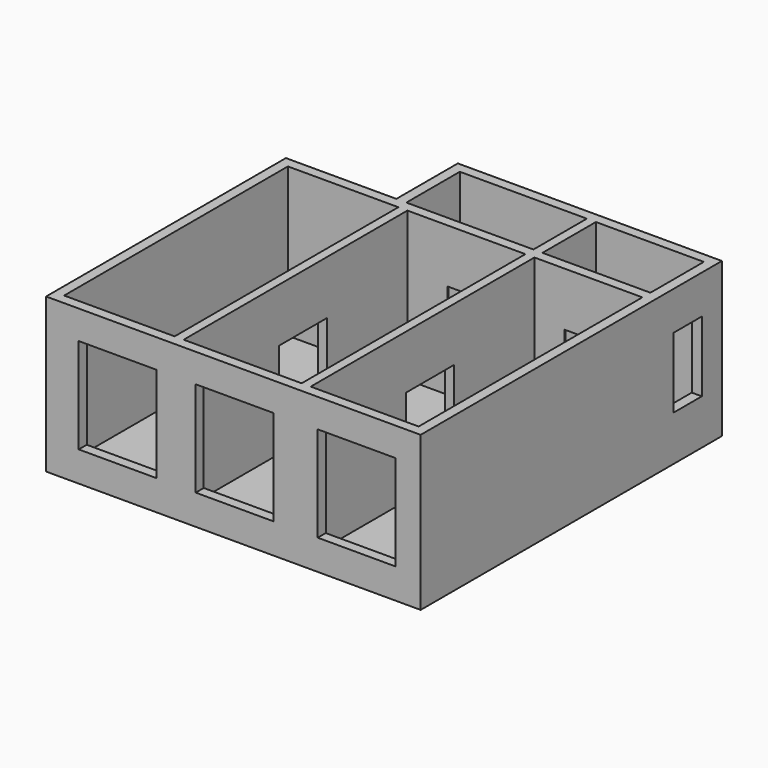
from build123d import *

# Parameters (mm, degrees)
F0_W           = 2200
F0_H           = 5570
F0_W_2         = 2350
F0_W_3         = 2150
F0_W_4         = 2530
F0_H_2         = 1330
F1_DEPTH       = 2970
F2_W           = 1550
F2_H           = 1900
F3_DEPTH       = 200
F4_W           = 700
F4_H           = 1400
F5_DEPTH       = 200
F7_DEPTH       = 100
F9_W           = 1200
F9_H           = 1900
F10_DEPTH      = 3000
F8_TEXT_SIZE   = 357.9835096995
F8_TEXT_SIZE_2 = 338.9626741409
F8_TEXT_SIZE_3 = 365.0618924035
F11_DEPTH      = 25
F12_W          = 800
F12_H          = 1900
F12_W_2        = 13.7615062607
F12_H_2        = 90.81533515
F12_W_3        = 16.1035829224
F12_H_3        = 106.2712360484
F12_H_4        = 150.8896411397
F13_DEPTH      = 25


# Not quite as in the source:
# - Text() gives the source's letters only with a copy of the font that has no kerning and outlines rounded to 1/6400 em; it was checked with that copy


with BuildPart() as f1:
    # F0 (on Top) → F1 (new body)
    with BuildSketch(Plane.XY):
        Polygon((200, 7300), (-5060, 7300), (-5060, 5770), (-7260, 5770), (-7260, -200), (200, -200), align=None)
        with Locations((-5960, 2785)):
            Rectangle(F0_W, F0_H, mode=Mode.SUBTRACT)
        with Locations((-3505, 2785)):
            Rectangle(F0_W_2, F0_H, mode=Mode.SUBTRACT)
        with Locations((-1075, 2785)):
            Rectangle(F0_W_3, F0_H, mode=Mode.SUBTRACT)
        with Locations((-3595, 6435)):
            Rectangle(F0_W_4, F0_H_2, mode=Mode.SUBTRACT)
        with Locations((-1075, 6435)):
            Rectangle(F0_W_3, F0_H_2, mode=Mode.SUBTRACT)
    extrude(amount=F1_DEPTH)

    # F2 (on face) → F3 (cut, through all)
    with BuildSketch(Plane(origin=(0, 0, 0), x_dir=(-1, 0, 0), z_dir=(0, 1, 0))):
        with Locations((1075, 1450)):
            Rectangle(F2_W, F2_H)
        with Locations((3505, 1450)):
            Rectangle(F2_W, F2_H)
        with Locations((5835, 1450)):
            Rectangle(F2_W, F2_H)
    extrude(amount=-F3_DEPTH, mode=Mode.SUBTRACT)

    # F4 (on face) → F5 (cut, through all)
    with BuildSketch(Plane(origin=(0, 0, 0), x_dir=(0, -1, 0), z_dir=(-1, 0, 0))):
        with Locations((-6450, 1500)):
            Rectangle(F4_W, F4_H)
    extrude(amount=-F5_DEPTH, mode=Mode.SUBTRACT)

    # F6 (on face) → F7 (join)
    with BuildSketch(Plane(origin=(0, 0, 0), x_dir=(1, 0, 0), z_dir=(0, 0, -1))):
        Polygon((200, 200), (-7260, 200), (-7260, -5770), (-5060, -5770), (-5060, -7300), (200, -7300), align=None)
    extrude(amount=F7_DEPTH)

    # F9 (on face) → F10 (cut)
    with BuildSketch(Plane(origin=(-4860, 0, 0), x_dir=(0, -1, 0), z_dir=(-1, 0, 0))):
        with Locations((-2970, 950)):
            Rectangle(F9_W, F9_H)
    extrude(amount=-F10_DEPTH, mode=Mode.SUBTRACT)

    # F8 (on face) → F11 (cut)
    with BuildSketch(Plane.XY):
        with Locations((-6638.8936042786, 3402.1844863892)):
            Text('Cuisine', F8_TEXT_SIZE, font='Open Sans', text_align=(TextAlign.LEFT, TextAlign.BOTTOM))
        with Locations((-6638.8936042786, 2915.3269131978)):
            Text('12m²', F8_TEXT_SIZE, font='Open Sans', text_align=(TextAlign.LEFT, TextAlign.BOTTOM))
        with Locations((-4455.9426307678, 3903.7611484528)):
            Text('salon', F8_TEXT_SIZE_2, font='Open Sans', text_align=(TextAlign.LEFT, TextAlign.BOTTOM))
        with Locations((-4455.9426307678, 3442.7719116211)):
            Text('12m²', F8_TEXT_SIZE_2, font='Open Sans', text_align=(TextAlign.LEFT, TextAlign.BOTTOM))
        with Locations((-4455.9426307678, 2520.7934379578)):
            Text('surface sans', F8_TEXT_SIZE_2, font='Open Sans', text_align=(TextAlign.LEFT, TextAlign.BOTTOM))
        with Locations((-4455.9426307678, 2059.8042011261)):
            Text('cloison 38m²', F8_TEXT_SIZE_2, font='Open Sans', text_align=(TextAlign.LEFT, TextAlign.BOTTOM))
        with Locations((-1840.2670621872, 3832.0169448853)):
            Text('chambre', F8_TEXT_SIZE_3, font='Open Sans', text_align=(TextAlign.LEFT, TextAlign.BOTTOM))
        with Locations((-1840.2670621872, 3335.5327712165)):
            Text('12m²', F8_TEXT_SIZE_3, font='Open Sans', text_align=(TextAlign.LEFT, TextAlign.BOTTOM))
    extrude(amount=-F11_DEPTH, mode=Mode.SUBTRACT)

    # F12 (on face) → F13 (cut)
    with BuildSketch(Plane.XZ.offset(-5570)):
        with Locations((-1150, 950)):
            Rectangle(F12_W, F12_H)
        with BuildLine():
            Line((-1405.2248319818, 966.460329377), (-1390.1375544051, 966.460329377))
            Line((-1390.1375544051, 966.460329377), (-1388.891329368, 964.5512186819))
            add(Edge.make_bspline(
                [(-1388.891329368, 964.5512186819), (-1391.0655943263, 956.2518902433), (-1395.1224545534, 945.2745037464)],
                knots=[0, 0, 0, 1, 1, 1], degree=2))
            add(Edge.make_bspline(
                [(-1395.1224545534, 945.2745037464), (-1399.1793147806, 934.2971172494), (-1403.5543601236, 924.8576254791)],
                knots=[0, 0, 0, 1, 1, 1], degree=2))
            Line((-1403.5543601236, 924.8576254791), (-1413.9218918151, 924.8576254791))
            add(Edge.make_bspline(
                [(-1413.9218918151, 924.8576254791), (-1411.6945960042, 933.4751390335), (-1409.0032802326, 946.149512815)],
                knots=[0, 0, 0, 1, 1, 1], degree=2))
            add(Edge.make_bspline(
                [(-1409.0032802326, 946.149512815), (-1406.311964461, 958.8238865965), (-1405.2248319818, 966.460329377)],
                knots=[0, 0, 0, 1, 1, 1], degree=2))
        make_face(mode=Mode.SUBTRACT)
        with BuildLine():
            add(Edge.make_bspline(
                [(-1442.5850676683, 1061.5313904515), (-1432.8008753558, 1053.4574431367), (-1432.8008753558, 1039.3777517602)],
                knots=[0, 0, 0, 1, 1, 1], degree=2))
            add(Edge.make_bspline(
                [(-1432.8008753558, 1039.3777517602), (-1432.8008753558, 1027.7639950315), (-1439.3104125176, 1020.3927065142)],
                knots=[0, 0, 0, 1, 1, 1], degree=2))
            add(Edge.make_bspline(
                [(-1439.3104125176, 1020.3927065142), (-1445.8199496795, 1013.0214179969), (-1457.751891524, 1010.5289679228)],
                knots=[0, 0, 0, 1, 1, 1], degree=2))
            Line((-1457.751891524, 1010.5289679228), (-1457.751891524, 1009.8660822647))
            add(Edge.make_bspline(
                [(-1457.751891524, 1009.8660822647), (-1443.1684070474, 1008.0630332749), (-1436.1285613591, 1000.5989407655)],
                knots=[0, 0, 0, 1, 1, 1], degree=2))
            add(Edge.make_bspline(
                [(-1436.1285613591, 1000.5989407655), (-1429.0887156708, 993.1348482561), (-1429.0887156708, 981.0438138536)],
                knots=[0, 0, 0, 1, 1, 1], degree=2))
            add(Edge.make_bspline(
                [(-1429.0887156708, 981.0438138536), (-1429.0887156708, 963.7292404659), (-1441.1002037943, 954.3958104009)],
                knots=[0, 0, 0, 1, 1, 1], degree=2))
            add(Edge.make_bspline(
                [(-1441.1002037943, 954.3958104009), (-1453.1116919178, 945.0623803358), (-1475.2255574697, 945.0623803358)],
                knots=[0, 0, 0, 1, 1, 1], degree=2))
            add(Edge.make_bspline(
                [(-1475.2255574697, 945.0623803358), (-1484.8506572242, 945.0623803358), (-1492.8450582601, 946.5207287835)],
                knots=[0, 0, 0, 1, 1, 1], degree=2))
            add(Edge.make_bspline(
                [(-1492.8450582601, 946.5207287835), (-1500.8394592959, 947.9790772311), (-1508.3698403711, 951.6116906371)],
                knots=[0, 0, 0, 1, 1, 1], degree=2))
            Line((-1508.3698403711, 951.6116906371), (-1508.3698403711, 964.7103112398))
            add(Edge.make_bspline(
                [(-1508.3698403711, 964.7103112398), (-1500.4947587537, 960.8125435706), (-1491.5855755098, 958.784113457)],
                knots=[0, 0, 0, 1, 1, 1], degree=2))
            add(Edge.make_bspline(
                [(-1491.5855755098, 958.784113457), (-1482.6763922659, 956.7556833434), (-1474.7217643696, 956.7556833434)],
                knots=[0, 0, 0, 1, 1, 1], degree=2))
            add(Edge.make_bspline(
                [(-1474.7217643696, 956.7556833434), (-1443.3274996053, 956.7556833434), (-1443.3274996053, 981.3619989695)],
                knots=[0, 0, 0, 1, 1, 1], degree=2))
            add(Edge.make_bspline(
                [(-1443.3274996053, 981.3619989695), (-1443.3274996053, 1003.4228336687), (-1477.9566463807, 1003.4228336687)],
                knots=[0, 0, 0, 1, 1, 1], degree=2))
            Line((-1477.9566463807, 1003.4228336687), (-1489.8885882253, 1003.4228336687))
            Line((-1489.8885882253, 1003.4228336687), (-1489.8885882253, 1015.2487138079))
            Line((-1489.8885882253, 1015.2487138079), (-1477.7975538228, 1015.2487138079))
            add(Edge.make_bspline(
                [(-1477.7975538228, 1015.2487138079), (-1463.6383161673, 1015.2487138079), (-1455.3522454419, 1021.5063544197)],
                knots=[0, 0, 0, 1, 1, 1], degree=2))
            add(Edge.make_bspline(
                [(-1455.3522454419, 1021.5063544197), (-1447.0661747166, 1027.7639950315), (-1447.0661747166, 1038.8739586601)],
                knots=[0, 0, 0, 1, 1, 1], degree=2))
            add(Edge.make_bspline(
                [(-1447.0661747166, 1038.8739586601), (-1447.0661747166, 1047.7301110514), (-1453.1514650573, 1052.7945574787)],
                knots=[0, 0, 0, 1, 1, 1], degree=2))
            add(Edge.make_bspline(
                [(-1453.1514650573, 1052.7945574787), (-1459.236755398, 1057.859003906), (-1469.6838333685, 1057.859003906)],
                knots=[0, 0, 0, 1, 1, 1], degree=2))
            add(Edge.make_bspline(
                [(-1469.6838333685, 1057.859003906), (-1477.6384612649, 1057.859003906), (-1484.6783069532, 1055.6979966609)],
                knots=[0, 0, 0, 1, 1, 1], degree=2))
            add(Edge.make_bspline(
                [(-1484.6783069532, 1055.6979966609), (-1491.7181526414, 1053.5369894157), (-1500.7599130169, 1047.7301110514)],
                knots=[0, 0, 0, 1, 1, 1], degree=2))
            Line((-1500.7599130169, 1047.7301110514), (-1507.7069547131, 1057.0105102638))
            add(Edge.make_bspline(
                [(-1507.7069547131, 1057.0105102638), (-1500.2561199168, 1062.8969349071), (-1490.524958457, 1066.2511363367)],
                knots=[0, 0, 0, 1, 1, 1], degree=2))
            add(Edge.make_bspline(
                [(-1490.524958457, 1066.2511363367), (-1480.7937969971, 1069.6053377663), (-1470.0020184844, 1069.6053377663)],
                knots=[0, 0, 0, 1, 1, 1], degree=2))
            add(Edge.make_bspline(
                [(-1470.0020184844, 1069.6053377663), (-1452.3692599808, 1069.6053377663), (-1442.5850676683, 1061.5313904515)],
                knots=[0, 0, 0, 1, 1, 1], degree=2))
        make_face(mode=Mode.SUBTRACT)
        with BuildLine():
            add(Edge.make_bspline(
                [(-1303.9624188613, 1061.5313904515), (-1294.1782265488, 1053.4574431367), (-1294.1782265488, 1039.3777517602)],
                knots=[0, 0, 0, 1, 1, 1], degree=2))
            add(Edge.make_bspline(
                [(-1294.1782265488, 1039.3777517602), (-1294.1782265488, 1027.7639950315), (-1300.6877637106, 1020.3927065142)],
                knots=[0, 0, 0, 1, 1, 1], degree=2))
            add(Edge.make_bspline(
                [(-1300.6877637106, 1020.3927065142), (-1307.1973008725, 1013.0214179969), (-1319.129242717, 1010.5289679228)],
                knots=[0, 0, 0, 1, 1, 1], degree=2))
            Line((-1319.129242717, 1010.5289679228), (-1319.129242717, 1009.8660822647))
            add(Edge.make_bspline(
                [(-1319.129242717, 1009.8660822647), (-1304.5457582403, 1008.0630332749), (-1297.5059125521, 1000.5989407655)],
                knots=[0, 0, 0, 1, 1, 1], degree=2))
            add(Edge.make_bspline(
                [(-1297.5059125521, 1000.5989407655), (-1290.4660668638, 993.1348482561), (-1290.4660668638, 981.0438138536)],
                knots=[0, 0, 0, 1, 1, 1], degree=2))
            add(Edge.make_bspline(
                [(-1290.4660668638, 981.0438138536), (-1290.4660668638, 963.7292404659), (-1302.4775549873, 954.3958104009)],
                knots=[0, 0, 0, 1, 1, 1], degree=2))
            add(Edge.make_bspline(
                [(-1302.4775549873, 954.3958104009), (-1314.4890431108, 945.0623803358), (-1336.6029086626, 945.0623803358)],
                knots=[0, 0, 0, 1, 1, 1], degree=2))
            add(Edge.make_bspline(
                [(-1336.6029086626, 945.0623803358), (-1346.2280084172, 945.0623803358), (-1354.222409453, 946.5207287835)],
                knots=[0, 0, 0, 1, 1, 1], degree=2))
            add(Edge.make_bspline(
                [(-1354.222409453, 946.5207287835), (-1362.2168104889, 947.9790772311), (-1369.7471915641, 951.6116906371)],
                knots=[0, 0, 0, 1, 1, 1], degree=2))
            Line((-1369.7471915641, 951.6116906371), (-1369.7471915641, 964.7103112398))
            add(Edge.make_bspline(
                [(-1369.7471915641, 964.7103112398), (-1361.8721099467, 960.8125435706), (-1352.9629267028, 958.784113457)],
                knots=[0, 0, 0, 1, 1, 1], degree=2))
            add(Edge.make_bspline(
                [(-1352.9629267028, 958.784113457), (-1344.0537434589, 956.7556833434), (-1336.0991155625, 956.7556833434)],
                knots=[0, 0, 0, 1, 1, 1], degree=2))
            add(Edge.make_bspline(
                [(-1336.0991155625, 956.7556833434), (-1304.7048507983, 956.7556833434), (-1304.7048507983, 981.3619989695)],
                knots=[0, 0, 0, 1, 1, 1], degree=2))
            add(Edge.make_bspline(
                [(-1304.7048507983, 981.3619989695), (-1304.7048507983, 1003.4228336687), (-1339.3339975737, 1003.4228336687)],
                knots=[0, 0, 0, 1, 1, 1], degree=2))
            Line((-1339.3339975737, 1003.4228336687), (-1351.2659394182, 1003.4228336687))
            Line((-1351.2659394182, 1003.4228336687), (-1351.2659394182, 1015.2487138079))
            Line((-1351.2659394182, 1015.2487138079), (-1339.1749050158, 1015.2487138079))
            add(Edge.make_bspline(
                [(-1339.1749050158, 1015.2487138079), (-1325.0156673603, 1015.2487138079), (-1316.7295966349, 1021.5063544197)],
                knots=[0, 0, 0, 1, 1, 1], degree=2))
            add(Edge.make_bspline(
                [(-1316.7295966349, 1021.5063544197), (-1308.4435259095, 1027.7639950315), (-1308.4435259095, 1038.8739586601)],
                knots=[0, 0, 0, 1, 1, 1], degree=2))
            add(Edge.make_bspline(
                [(-1308.4435259095, 1038.8739586601), (-1308.4435259095, 1047.7301110514), (-1314.5288162503, 1052.7945574787)],
                knots=[0, 0, 0, 1, 1, 1], degree=2))
            add(Edge.make_bspline(
                [(-1314.5288162503, 1052.7945574787), (-1320.614106591, 1057.859003906), (-1331.0611845615, 1057.859003906)],
                knots=[0, 0, 0, 1, 1, 1], degree=2))
            add(Edge.make_bspline(
                [(-1331.0611845615, 1057.859003906), (-1339.0158124578, 1057.859003906), (-1346.0556581461, 1055.6979966609)],
                knots=[0, 0, 0, 1, 1, 1], degree=2))
            add(Edge.make_bspline(
                [(-1346.0556581461, 1055.6979966609), (-1353.0955038344, 1053.5369894157), (-1362.1372642099, 1047.7301110514)],
                knots=[0, 0, 0, 1, 1, 1], degree=2))
            Line((-1362.1372642099, 1047.7301110514), (-1369.084305906, 1057.0105102638))
            add(Edge.make_bspline(
                [(-1369.084305906, 1057.0105102638), (-1361.6334711098, 1062.8969349071), (-1351.9023096499, 1066.2511363367)],
                knots=[0, 0, 0, 1, 1, 1], degree=2))
            add(Edge.make_bspline(
                [(-1351.9023096499, 1066.2511363367), (-1342.1711481901, 1069.6053377663), (-1331.3793696774, 1069.6053377663)],
                knots=[0, 0, 0, 1, 1, 1], degree=2))
            add(Edge.make_bspline(
                [(-1331.3793696774, 1069.6053377663), (-1313.7466111738, 1069.6053377663), (-1303.9624188613, 1061.5313904515)],
                knots=[0, 0, 0, 1, 1, 1], degree=2))
        make_face(mode=Mode.SUBTRACT)
        with BuildLine():
            Line((-1136.4379553642, 946.732852194), (-1150.1729461985, 946.732852194))
            Line((-1150.1729461985, 946.732852194), (-1150.1729461985, 1005.8092220376))
            add(Edge.make_bspline(
                [(-1150.1729461985, 1005.8092220376), (-1150.1729461985, 1016.6805468293), (-1154.8131458047, 1022.1029515119)],
                knots=[0, 0, 0, 1, 1, 1], degree=2))
            add(Edge.make_bspline(
                [(-1154.8131458047, 1022.1029515119), (-1159.4533454109, 1027.5253561946), (-1169.2375377234, 1027.5253561946)],
                knots=[0, 0, 0, 1, 1, 1], degree=2))
            add(Edge.make_bspline(
                [(-1169.2375377234, 1027.5253561946), (-1182.0710040629, 1027.5253561946), (-1188.2093252562, 1020.1540676773)],
                knots=[0, 0, 0, 1, 1, 1], degree=2))
            add(Edge.make_bspline(
                [(-1188.2093252562, 1020.1540676773), (-1194.3476464496, 1012.7827791601), (-1194.3476464496, 997.4568627464)],
                knots=[0, 0, 0, 1, 1, 1], degree=2))
            Line((-1194.3476464496, 997.4568627464), (-1194.3476464496, 946.732852194))
            Line((-1194.3476464496, 946.732852194), (-1208.1091527103, 946.732852194))
            Line((-1208.1091527103, 946.732852194), (-1208.1091527103, 1005.8092220376))
            add(Edge.make_bspline(
                [(-1208.1091527103, 1005.8092220376), (-1208.1091527103, 1016.6805468293), (-1212.7493523165, 1022.1029515119)],
                knots=[0, 0, 0, 1, 1, 1], degree=2))
            add(Edge.make_bspline(
                [(-1212.7493523165, 1022.1029515119), (-1217.3895519227, 1027.5253561946), (-1227.2532905142, 1027.5253561946)],
                knots=[0, 0, 0, 1, 1, 1], degree=2))
            add(Edge.make_bspline(
                [(-1227.2532905142, 1027.5253561946), (-1240.1663031326, 1027.5253561946), (-1246.1720471943, 1019.7828517088)],
                knots=[0, 0, 0, 1, 1, 1], degree=2))
            add(Edge.make_bspline(
                [(-1246.1720471943, 1019.7828517088), (-1252.177791256, 1012.0403472231), (-1252.177791256, 994.3810732932)],
                knots=[0, 0, 0, 1, 1, 1], degree=2))
            Line((-1252.177791256, 994.3810732932), (-1252.177791256, 946.732852194))
            Line((-1252.177791256, 946.732852194), (-1265.9392975167, 946.732852194))
            Line((-1265.9392975167, 946.732852194), (-1265.9392975167, 1037.548187344))
            Line((-1265.9392975167, 1037.548187344), (-1254.7497876092, 1037.548187344))
            Line((-1254.7497876092, 1037.548187344), (-1252.5224917982, 1025.1124523994))
            Line((-1252.5224917982, 1025.1124523994), (-1251.8596061402, 1025.1124523994))
            add(Edge.make_bspline(
                [(-1251.8596061402, 1025.1124523994), (-1247.961838471, 1031.7413089797), (-1240.8689619301, 1035.479984091)],
                knots=[0, 0, 0, 1, 1, 1], degree=2))
            add(Edge.make_bspline(
                [(-1240.8689619301, 1035.479984091), (-1233.7760853892, 1039.2186592023), (-1224.9994792769, 1039.2186592023)],
                knots=[0, 0, 0, 1, 1, 1], degree=2))
            add(Edge.make_bspline(
                [(-1224.9994792769, 1039.2186592023), (-1203.707591941, 1039.2186592023), (-1197.1582816396, 1023.7866810833)],
                knots=[0, 0, 0, 1, 1, 1], degree=2))
            Line((-1197.1582816396, 1023.7866810833), (-1196.4953959816, 1023.7866810833))
            add(Edge.make_bspline(
                [(-1196.4953959816, 1023.7866810833), (-1192.4385357545, 1030.9193307637), (-1184.7358044082, 1035.068994983)],
                knots=[0, 0, 0, 1, 1, 1], degree=2))
            add(Edge.make_bspline(
                [(-1184.7358044082, 1035.068994983), (-1177.0330730619, 1039.2186592023), (-1167.1693344704, 1039.2186592023)],
                knots=[0, 0, 0, 1, 1, 1], degree=2))
            add(Edge.make_bspline(
                [(-1167.1693344704, 1039.2186592023), (-1151.7638717778, 1039.2186592023), (-1144.100913571, 1031.3038044454)],
                knots=[0, 0, 0, 1, 1, 1], degree=2))
            add(Edge.make_bspline(
                [(-1144.100913571, 1031.3038044454), (-1136.4379553642, 1023.3889496885), (-1136.4379553642, 1005.9683145955)],
                knots=[0, 0, 0, 1, 1, 1], degree=2))
            Line((-1136.4379553642, 1005.9683145955), (-1136.4379553642, 946.732852194))
        make_face(mode=Mode.SUBTRACT)
        with BuildLine():
            Line((-1068.558463982, 1005.1463363796), (-1068.558463982, 995.2825977881))
            Line((-1068.558463982, 995.2825977881), (-1118.6195888764, 995.2825977881))
            Line((-1118.6195888764, 995.2825977881), (-1118.6195888764, 1003.9001113425))
            Line((-1118.6195888764, 1003.9001113425), (-1099.0512042513, 1022.9647028674))
            add(Edge.make_bspline(
                [(-1099.0512042513, 1022.9647028674), (-1091.679915734, 1030.0973525478), (-1088.2859411649, 1034.1144396354)],
                knots=[0, 0, 0, 1, 1, 1], degree=2))
            add(Edge.make_bspline(
                [(-1088.2859411649, 1034.1144396354), (-1084.8919665958, 1038.1315267231), (-1083.5264221403, 1041.2736047421)],
                knots=[0, 0, 0, 1, 1, 1], degree=2))
            add(Edge.make_bspline(
                [(-1083.5264221403, 1041.2736047421), (-1082.1608776848, 1044.4156827612), (-1082.1608776848, 1048.8967898095)],
                knots=[0, 0, 0, 1, 1, 1], degree=2))
            add(Edge.make_bspline(
                [(-1082.1608776848, 1048.8967898095), (-1082.1608776848, 1054.5445756159), (-1085.4753059749, 1057.3949839454)],
                knots=[0, 0, 0, 1, 1, 1], degree=2))
            add(Edge.make_bspline(
                [(-1085.4753059749, 1057.3949839454), (-1088.789734265, 1060.2453922749), (-1094.0132732503, 1060.2453922749)],
                knots=[0, 0, 0, 1, 1, 1], degree=2))
            add(Edge.make_bspline(
                [(-1094.0132732503, 1060.2453922749), (-1098.3087723143, 1060.2453922749), (-1102.3656325415, 1058.680982122)],
                knots=[0, 0, 0, 1, 1, 1], degree=2))
            add(Edge.make_bspline(
                [(-1102.3656325415, 1058.680982122), (-1106.4224927686, 1057.116571969), (-1112.149824854, 1052.9536500366)],
                knots=[0, 0, 0, 1, 1, 1], degree=2))
            Line((-1112.149824854, 1052.9536500366), (-1117.6120026761, 1060.2453922749))
            add(Edge.make_bspline(
                [(-1117.6120026761, 1060.2453922749), (-1106.7671933108, 1069.4462452084), (-1094.1723658082, 1069.4462452084)],
                knots=[0, 0, 0, 1, 1, 1], degree=2))
            add(Edge.make_bspline(
                [(-1094.1723658082, 1069.4462452084), (-1083.2214947376, 1069.4462452084), (-1077.1362043969, 1064.0636136652)],
                knots=[0, 0, 0, 1, 1, 1], degree=2))
            add(Edge.make_bspline(
                [(-1077.1362043969, 1064.0636136652), (-1071.0509140562, 1058.680982122), (-1071.0509140562, 1049.4005829096)],
                knots=[0, 0, 0, 1, 1, 1], degree=2))
            add(Edge.make_bspline(
                [(-1071.0509140562, 1049.4005829096), (-1071.0509140562, 1042.7717263293), (-1074.7365583148, 1036.5140857175)],
                knots=[0, 0, 0, 1, 1, 1], degree=2))
            add(Edge.make_bspline(
                [(-1074.7365583148, 1036.5140857175), (-1078.4222025735, 1030.2564451057), (-1090.6192986812, 1018.8282963613)],
                knots=[0, 0, 0, 1, 1, 1], degree=2))
            Line((-1090.6192986812, 1018.8282963613), (-1105.0171751736, 1005.1463363796))
            Line((-1105.0171751736, 1005.1463363796), (-1068.558463982, 1005.1463363796))
        make_face(mode=Mode.SUBTRACT)
        with BuildLine():
            add(Edge.make_bspline(
                [(-1487.8203849722, 1256.247423641), (-1478.221800644, 1269.8233219174), (-1459.316301677, 1269.8233219174)],
                knots=[0, 0, 0, 1, 1, 1], degree=2))
            add(Edge.make_bspline(
                [(-1459.316301677, 1269.8233219174), (-1441.4183889102, 1269.8233219174), (-1431.5148771792, 1257.5997103833)],
                knots=[0, 0, 0, 1, 1, 1], degree=2))
            add(Edge.make_bspline(
                [(-1431.5148771792, 1257.5997103833), (-1421.6113654483, 1245.3760988493), (-1421.6113654483, 1223.0235944606)],
                knots=[0, 0, 0, 1, 1, 1], degree=2))
            add(Edge.make_bspline(
                [(-1421.6113654483, 1223.0235944606), (-1421.6113654483, 1200.6445746455), (-1431.5944234582, 1188.2486128403)],
                knots=[0, 0, 0, 1, 1, 1], degree=2))
            add(Edge.make_bspline(
                [(-1431.5944234582, 1188.2486128403), (-1441.5774814681, 1175.8526510352), (-1459.316301677, 1175.8526510352)],
                knots=[0, 0, 0, 1, 1, 1], degree=2))
            add(Edge.make_bspline(
                [(-1459.316301677, 1175.8526510352), (-1468.1989694946, 1175.8526510352), (-1475.5304848724, 1179.1273061859)],
                knots=[0, 0, 0, 1, 1, 1], degree=2))
            add(Edge.make_bspline(
                [(-1475.5304848724, 1179.1273061859), (-1482.8620002502, 1182.4019613365), (-1487.8203849722, 1189.2164259011)],
                knots=[0, 0, 0, 1, 1, 1], degree=2))
            Line((-1487.8203849722, 1189.2164259011), (-1488.8279711724, 1189.2164259011))
            Line((-1488.8279711724, 1189.2164259011), (-1491.7181526414, 1177.5231228934))
            Line((-1491.7181526414, 1177.5231228934), (-1501.5818912329, 1177.5231228934))
            Line((-1501.5818912329, 1177.5231228934), (-1501.5818912329, 1306.4676410933))
            Line((-1501.5818912329, 1306.4676410933), (-1487.8203849722, 1306.4676410933))
            Line((-1487.8203849722, 1306.4676410933), (-1487.8203849722, 1275.1264071816))
            add(Edge.make_bspline(
                [(-1487.8203849722, 1275.1264071816), (-1487.8203849722, 1264.5997829321), (-1488.4832706302, 1256.247423641)],
                knots=[0, 0, 0, 1, 1, 1], degree=2))
            Line((-1488.4832706302, 1256.247423641), (-1487.8203849722, 1256.247423641))
        make_face(mode=Mode.SUBTRACT)
        with BuildLine():
            Line((-1331.5384622353, 1177.5231228934), (-1341.7469013689, 1177.5231228934))
            Line((-1341.7469013689, 1177.5231228934), (-1344.47799028, 1190.4626509382))
            Line((-1344.47799028, 1190.4626509382), (-1345.140875938, 1190.4626509382))
            add(Edge.make_bspline(
                [(-1345.140875938, 1190.4626509382), (-1351.9288250763, 1181.9246836628), (-1358.677001075, 1178.888667349)],
                knots=[0, 0, 0, 1, 1, 1], degree=2))
            add(Edge.make_bspline(
                [(-1358.677001075, 1178.888667349), (-1365.4251770737, 1175.8526510352), (-1375.5540699284, 1175.8526510352)],
                knots=[0, 0, 0, 1, 1, 1], degree=2))
            add(Edge.make_bspline(
                [(-1375.5540699284, 1175.8526510352), (-1389.0504219259, 1175.8526510352), (-1396.7133801327, 1182.8262081577)],
                knots=[0, 0, 0, 1, 1, 1], degree=2))
            add(Edge.make_bspline(
                [(-1396.7133801327, 1182.8262081577), (-1404.3763383395, 1189.7997652801), (-1404.3763383395, 1202.6332316196)],
                knots=[0, 0, 0, 1, 1, 1], degree=2))
            add(Edge.make_bspline(
                [(-1404.3763383395, 1202.6332316196), (-1404.3763383395, 1230.1297287146), (-1360.3872460727, 1231.4555000307)],
                knots=[0, 0, 0, 1, 1, 1], degree=2))
            Line((-1360.3872460727, 1231.4555000307), (-1344.9817833801, 1231.9592931308))
            Line((-1344.9817833801, 1231.9592931308), (-1344.9817833801, 1237.6070789372))
            add(Edge.make_bspline(
                [(-1344.9817833801, 1237.6070789372), (-1344.9817833801, 1248.2927957446), (-1349.5689521337, 1253.3837575983)],
                knots=[0, 0, 0, 1, 1, 1], degree=2))
            add(Edge.make_bspline(
                [(-1349.5689521337, 1253.3837575983), (-1354.1561208872, 1258.4747194519), (-1364.2850137419, 1258.4747194519)],
                knots=[0, 0, 0, 1, 1, 1], degree=2))
            add(Edge.make_bspline(
                [(-1364.2850137419, 1258.4747194519), (-1375.6336162074, 1258.4747194519), (-1389.9519464208, 1251.5276777558)],
                knots=[0, 0, 0, 1, 1, 1], degree=2))
            Line((-1389.9519464208, 1251.5276777558), (-1394.1944146322, 1262.0543020053))
            add(Edge.make_bspline(
                [(-1394.1944146322, 1262.0543020053), (-1387.4860117729, 1265.6869154113), (-1379.4916107371, 1267.7551186644)],
                knots=[0, 0, 0, 1, 1, 1], degree=2))
            add(Edge.make_bspline(
                [(-1379.4916107371, 1267.7551186644), (-1371.4972097013, 1269.8233219174), (-1363.4365200996, 1269.8233219174)],
                knots=[0, 0, 0, 1, 1, 1], degree=2))
            add(Edge.make_bspline(
                [(-1363.4365200996, 1269.8233219174), (-1347.2090791911, 1269.8233219174), (-1339.3737707132, 1262.6243836712)],
                knots=[0, 0, 0, 1, 1, 1], degree=2))
            add(Edge.make_bspline(
                [(-1339.3737707132, 1262.6243836712), (-1331.5384622353, 1255.425445425), (-1331.5384622353, 1239.5161896323)],
                knots=[0, 0, 0, 1, 1, 1], degree=2))
            Line((-1331.5384622353, 1239.5161896323), (-1331.5384622353, 1177.5231228934))
        make_face(mode=Mode.SUBTRACT)
        with Locations((-1296.3392337939, 1222.9307904684)):
            Rectangle(F12_W_2, F12_H_2, mode=Mode.SUBTRACT)
        with BuildLine():
            Line((-1217.3630364964, 1268.3384580434), (-1185.9687717321, 1268.3384580434))
            Line((-1185.9687717321, 1268.3384580434), (-1185.9687717321, 1259.6413982101))
            Line((-1185.9687717321, 1259.6413982101), (-1202.7795520197, 1257.652741236))
            add(Edge.make_bspline(
                [(-1202.7795520197, 1257.652741236), (-1200.4727099298, 1254.762559767), (-1198.6431455136, 1250.0693293081)],
                knots=[0, 0, 0, 1, 1, 1], degree=2))
            add(Edge.make_bspline(
                [(-1198.6431455136, 1250.0693293081), (-1196.8135810975, 1245.3760988493), (-1196.8135810975, 1239.5161896323)],
                knots=[0, 0, 0, 1, 1, 1], degree=2))
            add(Edge.make_bspline(
                [(-1196.8135810975, 1239.5161896323), (-1196.8135810975, 1226.1524147665), (-1205.9348877519, 1218.1977868701)],
                knots=[0, 0, 0, 1, 1, 1], degree=2))
            add(Edge.make_bspline(
                [(-1205.9348877519, 1218.1977868701), (-1215.0561944064, 1210.2431589738), (-1230.9654501991, 1210.2431589738)],
                knots=[0, 0, 0, 1, 1, 1], degree=2))
            add(Edge.make_bspline(
                [(-1230.9654501991, 1210.2431589738), (-1235.0223104263, 1210.2431589738), (-1238.5753775533, 1210.9060446318)],
                knots=[0, 0, 0, 1, 1, 1], degree=2))
            add(Edge.make_bspline(
                [(-1238.5753775533, 1210.9060446318), (-1247.3519836656, 1206.2658450256), (-1247.3519836656, 1199.2392570505)],
                knots=[0, 0, 0, 1, 1, 1], degree=2))
            add(Edge.make_bspline(
                [(-1247.3519836656, 1199.2392570505), (-1247.3519836656, 1195.5005819392), (-1244.2894519255, 1193.7240483757)],
                knots=[0, 0, 0, 1, 1, 1], degree=2))
            add(Edge.make_bspline(
                [(-1244.2894519255, 1193.7240483757), (-1241.2269201854, 1191.9475148122), (-1233.7760853892, 1191.9475148122)],
                knots=[0, 0, 0, 1, 1, 1], degree=2))
            Line((-1233.7760853892, 1191.9475148122), (-1217.7077370385, 1191.9475148122))
            add(Edge.make_bspline(
                [(-1217.7077370385, 1191.9475148122), (-1202.9386445776, 1191.9475148122), (-1195.0370475339, 1185.7296473398)],
                knots=[0, 0, 0, 1, 1, 1], degree=2))
            add(Edge.make_bspline(
                [(-1195.0370475339, 1185.7296473398), (-1187.1354504902, 1179.5117798675), (-1187.1354504902, 1167.659384302)],
                knots=[0, 0, 0, 1, 1, 1], degree=2))
            add(Edge.make_bspline(
                [(-1187.1354504902, 1167.659384302), (-1187.1354504902, 1152.5721067252), (-1199.2264848927, 1144.6572519684)],
                knots=[0, 0, 0, 1, 1, 1], degree=2))
            add(Edge.make_bspline(
                [(-1199.2264848927, 1144.6572519684), (-1211.3175192951, 1136.7423972115), (-1234.5185173261, 1136.7423972115)],
                knots=[0, 0, 0, 1, 1, 1], degree=2))
            add(Edge.make_bspline(
                [(-1234.5185173261, 1136.7423972115), (-1252.336883814, 1136.7423972115), (-1261.9884989949, 1143.3712537918)],
                knots=[0, 0, 0, 1, 1, 1], degree=2))
            add(Edge.make_bspline(
                [(-1261.9884989949, 1143.3712537918), (-1271.6401141758, 1150.0001103721), (-1271.6401141758, 1162.1176602008)],
                knots=[0, 0, 0, 1, 1, 1], degree=2))
            add(Edge.make_bspline(
                [(-1271.6401141758, 1162.1176602008), (-1271.6401141758, 1170.390473213), (-1266.3370289115, 1176.4492481274)],
                knots=[0, 0, 0, 1, 1, 1], degree=2))
            add(Edge.make_bspline(
                [(-1266.3370289115, 1176.4492481274), (-1261.0339436473, 1182.5080230418), (-1251.4353593191, 1184.6557725738)],
                knots=[0, 0, 0, 1, 1, 1], degree=2))
            add(Edge.make_bspline(
                [(-1251.4353593191, 1184.6557725738), (-1254.9088801671, 1186.2201827268), (-1257.2687531097, 1189.5346110169)],
                knots=[0, 0, 0, 1, 1, 1], degree=2))
            add(Edge.make_bspline(
                [(-1257.2687531097, 1189.5346110169), (-1259.6286260523, 1192.8490393071), (-1259.6286260523, 1197.2506000764)],
                knots=[0, 0, 0, 1, 1, 1], degree=2))
            add(Edge.make_bspline(
                [(-1259.6286260523, 1197.2506000764), (-1259.6286260523, 1202.2089847984), (-1256.9770834202, 1205.9476599097)],
                knots=[0, 0, 0, 1, 1, 1], degree=2))
            add(Edge.make_bspline(
                [(-1256.9770834202, 1205.9476599097), (-1254.3255407881, 1209.686335021), (-1248.5982087027, 1213.1598558691)],
                knots=[0, 0, 0, 1, 1, 1], degree=2))
            add(Edge.make_bspline(
                [(-1248.5982087027, 1213.1598558691), (-1255.6513121041, 1216.0500373381), (-1260.0793882998, 1223.0103367474)],
                knots=[0, 0, 0, 1, 1, 1], degree=2))
            add(Edge.make_bspline(
                [(-1260.0793882998, 1223.0103367474), (-1264.5074644954, 1229.9706361567), (-1264.5074644954, 1238.9328502533)],
                knots=[0, 0, 0, 1, 1, 1], degree=2))
            add(Edge.make_bspline(
                [(-1264.5074644954, 1238.9328502533), (-1264.5074644954, 1253.8345198457), (-1255.558508112, 1261.9217248737)],
                knots=[0, 0, 0, 1, 1, 1], degree=2))
            add(Edge.make_bspline(
                [(-1255.558508112, 1261.9217248737), (-1246.6095517286, 1270.0089299017), (-1230.2230182621, 1270.0089299017)],
                knots=[0, 0, 0, 1, 1, 1], degree=2))
            add(Edge.make_bspline(
                [(-1230.2230182621, 1270.0089299017), (-1223.0903685817, 1270.0089299017), (-1217.3630364964, 1268.3384580434)],
                knots=[0, 0, 0, 1, 1, 1], degree=2))
        make_face(mode=Mode.SUBTRACT)
        with BuildLine():
            add(Edge.make_bspline(
                [(-1302.0665658793, 1286.0242473996), (-1304.3866656824, 1288.3045740633), (-1304.3866656824, 1292.9447736695)],
                knots=[0, 0, 0, 1, 1, 1], degree=2))
            add(Edge.make_bspline(
                [(-1304.3866656824, 1292.9447736695), (-1304.3866656824, 1297.6645195546), (-1302.0665658793, 1299.8652999393)],
                knots=[0, 0, 0, 1, 1, 1], degree=2))
            add(Edge.make_bspline(
                [(-1302.0665658793, 1299.8652999393), (-1299.7464660762, 1302.0660803239), (-1296.2464298018, 1302.0660803239)],
                knots=[0, 0, 0, 1, 1, 1], degree=2))
            add(Edge.make_bspline(
                [(-1296.2464298018, 1302.0660803239), (-1292.9320015117, 1302.0660803239), (-1290.5323554296, 1299.8255267998)],
                knots=[0, 0, 0, 1, 1, 1], degree=2))
            add(Edge.make_bspline(
                [(-1290.5323554296, 1299.8255267998), (-1288.1327093475, 1297.5849732757), (-1288.1327093475, 1292.9447736695)],
                knots=[0, 0, 0, 1, 1, 1], degree=2))
            add(Edge.make_bspline(
                [(-1288.1327093475, 1292.9447736695), (-1288.1327093475, 1288.3045740633), (-1290.5323554296, 1286.0242473996)],
                knots=[0, 0, 0, 1, 1, 1], degree=2))
            add(Edge.make_bspline(
                [(-1290.5323554296, 1286.0242473996), (-1292.9320015117, 1283.743920736), (-1296.2464298018, 1283.743920736)],
                knots=[0, 0, 0, 1, 1, 1], degree=2))
            add(Edge.make_bspline(
                [(-1296.2464298018, 1283.743920736), (-1299.7464660762, 1283.743920736), (-1302.0665658793, 1286.0242473996)],
                knots=[0, 0, 0, 1, 1, 1], degree=2))
        make_face(mode=Mode.SUBTRACT)
        with BuildLine():
            Line((-1091.4147614708, 1177.5231228934), (-1105.1762677315, 1177.5231228934))
            Line((-1105.1762677315, 1177.5231228934), (-1105.1762677315, 1236.2813076211))
            add(Edge.make_bspline(
                [(-1105.1762677315, 1236.2813076211), (-1105.1762677315, 1247.3647558234), (-1110.2274564457, 1252.8401913587)],
                knots=[0, 0, 0, 1, 1, 1], degree=2))
            add(Edge.make_bspline(
                [(-1110.2274564457, 1252.8401913587), (-1115.2786451599, 1258.315626894), (-1126.0704236726, 1258.315626894)],
                knots=[0, 0, 0, 1, 1, 1], degree=2))
            add(Edge.make_bspline(
                [(-1126.0704236726, 1258.315626894), (-1140.3092076071, 1258.315626894), (-1146.9380641874, 1250.6128955477)],
                knots=[0, 0, 0, 1, 1, 1], degree=2))
            add(Edge.make_bspline(
                [(-1146.9380641874, 1250.6128955477), (-1153.5669207676, 1242.9101642014), (-1153.5669207676, 1225.1713439926)],
                knots=[0, 0, 0, 1, 1, 1], degree=2))
            Line((-1153.5669207676, 1225.1713439926), (-1153.5669207676, 1177.5231228934))
            Line((-1153.5669207676, 1177.5231228934), (-1167.3284270283, 1177.5231228934))
            Line((-1167.3284270283, 1177.5231228934), (-1167.3284270283, 1268.3384580434))
            Line((-1167.3284270283, 1268.3384580434), (-1156.1389171208, 1268.3384580434))
            Line((-1156.1389171208, 1268.3384580434), (-1153.9116213098, 1255.9027230988))
            Line((-1153.9116213098, 1255.9027230988), (-1153.2487356518, 1255.9027230988))
            add(Edge.make_bspline(
                [(-1153.2487356518, 1255.9027230988), (-1149.0062674404, 1262.611125958), (-1141.3830823731, 1266.3100279299)],
                knots=[0, 0, 0, 1, 1, 1], degree=2))
            add(Edge.make_bspline(
                [(-1141.3830823731, 1266.3100279299), (-1133.7598973057, 1270.0089299017), (-1124.3999518144, 1270.0089299017)],
                knots=[0, 0, 0, 1, 1, 1], degree=2))
            add(Edge.make_bspline(
                [(-1124.3999518144, 1270.0089299017), (-1107.9869029216, 1270.0089299017), (-1099.7008321962, 1262.0940751448)],
                knots=[0, 0, 0, 1, 1, 1], degree=2))
            add(Edge.make_bspline(
                [(-1099.7008321962, 1262.0940751448), (-1091.4147614708, 1254.1792203879), (-1091.4147614708, 1236.7585852949)],
                knots=[0, 0, 0, 1, 1, 1], degree=2))
            Line((-1091.4147614708, 1236.7585852949), (-1091.4147614708, 1177.5231228934))
        make_face(mode=Mode.SUBTRACT)
        with BuildLine():
            add(Edge.make_bspline(
                [(-996.0255152805, 1257.321298407), (-984.7962322334, 1244.6336669123), (-984.7962322334, 1223.0235944606)],
                knots=[0, 0, 0, 1, 1, 1], degree=2))
            add(Edge.make_bspline(
                [(-984.7962322334, 1223.0235944606), (-984.7962322334, 1200.8036672034), (-995.9724844278, 1188.3281591193)],
                knots=[0, 0, 0, 1, 1, 1], degree=2))
            add(Edge.make_bspline(
                [(-995.9724844278, 1188.3281591193), (-1007.1487366222, 1175.8526510352), (-1026.8762138051, 1175.8526510352)],
                knots=[0, 0, 0, 1, 1, 1], degree=2))
            add(Edge.make_bspline(
                [(-1026.8762138051, 1175.8526510352), (-1039.0733099129, 1175.8526510352), (-1048.5128016832, 1181.5799831206)],
                knots=[0, 0, 0, 1, 1, 1], degree=2))
            add(Edge.make_bspline(
                [(-1048.5128016832, 1181.5799831206), (-1057.9522934535, 1187.3073152059), (-1063.0962861598, 1197.9930320134)],
                knots=[0, 0, 0, 1, 1, 1], degree=2))
            add(Edge.make_bspline(
                [(-1063.0962861598, 1197.9930320134), (-1068.2402788661, 1208.6787488208), (-1068.2402788661, 1223.0235944606)],
                knots=[0, 0, 0, 1, 1, 1], degree=2))
            add(Edge.make_bspline(
                [(-1068.2402788661, 1223.0235944606), (-1068.2402788661, 1245.2170062914), (-1057.1303152376, 1257.6129680965)],
                knots=[0, 0, 0, 1, 1, 1], degree=2))
            add(Edge.make_bspline(
                [(-1057.1303152376, 1257.6129680965), (-1046.020351609, 1270.0089299017), (-1026.2928744261, 1270.0089299017)],
                knots=[0, 0, 0, 1, 1, 1], degree=2))
            add(Edge.make_bspline(
                [(-1026.2928744261, 1270.0089299017), (-1007.2547983275, 1270.0089299017), (-996.0255152805, 1257.321298407)],
                knots=[0, 0, 0, 1, 1, 1], degree=2))
        make_face(mode=Mode.SUBTRACT)
        with Locations((-953.7864411508, 1222.9307904684)):
            Rectangle(F12_W_2, F12_H_2, mode=Mode.SUBTRACT)
        with BuildLine():
            add(Edge.make_bspline(
                [(-959.5137732362, 1286.0242473996), (-961.8338730393, 1288.3045740633), (-961.8338730393, 1292.9447736695)],
                knots=[0, 0, 0, 1, 1, 1], degree=2))
            add(Edge.make_bspline(
                [(-961.8338730393, 1292.9447736695), (-961.8338730393, 1297.6645195546), (-959.5137732362, 1299.8652999393)],
                knots=[0, 0, 0, 1, 1, 1], degree=2))
            add(Edge.make_bspline(
                [(-959.5137732362, 1299.8652999393), (-957.1936734331, 1302.0660803239), (-953.6936371587, 1302.0660803239)],
                knots=[0, 0, 0, 1, 1, 1], degree=2))
            add(Edge.make_bspline(
                [(-953.6936371587, 1302.0660803239), (-950.3792088686, 1302.0660803239), (-947.9795627865, 1299.8255267998)],
                knots=[0, 0, 0, 1, 1, 1], degree=2))
            add(Edge.make_bspline(
                [(-947.9795627865, 1299.8255267998), (-945.5799167044, 1297.5849732757), (-945.5799167044, 1292.9447736695)],
                knots=[0, 0, 0, 1, 1, 1], degree=2))
            add(Edge.make_bspline(
                [(-945.5799167044, 1292.9447736695), (-945.5799167044, 1288.3045740633), (-947.9795627865, 1286.0242473996)],
                knots=[0, 0, 0, 1, 1, 1], degree=2))
            add(Edge.make_bspline(
                [(-947.9795627865, 1286.0242473996), (-950.3792088686, 1283.743920736), (-953.6936371587, 1283.743920736)],
                knots=[0, 0, 0, 1, 1, 1], degree=2))
            add(Edge.make_bspline(
                [(-953.6936371587, 1283.743920736), (-957.1936734331, 1283.743920736), (-959.5137732362, 1286.0242473996)],
                knots=[0, 0, 0, 1, 1, 1], degree=2))
        make_face(mode=Mode.SUBTRACT)
        with BuildLine():
            add(Edge.make_bspline(
                [(-891.9657246831, 1265.1963800244), (-884.8330750027, 1270.0089299017), (-876.2951077272, 1270.0089299017)],
                knots=[0, 0, 0, 1, 1, 1], degree=2))
            add(Edge.make_bspline(
                [(-876.2951077272, 1270.0089299017), (-870.249590526, 1270.0089299017), (-865.4502983619, 1269.0013437014)],
                knots=[0, 0, 0, 1, 1, 1], degree=2))
            Line((-865.4502983619, 1269.0013437014), (-867.359409057, 1256.247423641))
            add(Edge.make_bspline(
                [(-867.359409057, 1256.247423641), (-872.9806794371, 1257.4936486781), (-877.3026939275, 1257.4936486781)],
                knots=[0, 0, 0, 1, 1, 1], degree=2))
            add(Edge.make_bspline(
                [(-877.3026939275, 1257.4936486781), (-888.3331112771, 1257.4936486781), (-896.1551620418, 1248.5446922947)],
                knots=[0, 0, 0, 1, 1, 1], degree=2))
            add(Edge.make_bspline(
                [(-896.1551620418, 1248.5446922947), (-903.9772128065, 1239.5957359113), (-903.9772128065, 1226.2584764717)],
                knots=[0, 0, 0, 1, 1, 1], degree=2))
            Line((-903.9772128065, 1226.2584764717), (-903.9772128065, 1177.5231228934))
            Line((-903.9772128065, 1177.5231228934), (-917.7387190672, 1177.5231228934))
            Line((-917.7387190672, 1177.5231228934), (-917.7387190672, 1268.3384580434))
            Line((-917.7387190672, 1268.3384580434), (-906.3901166018, 1268.3384580434))
            Line((-906.3901166018, 1268.3384580434), (-904.7991910225, 1251.5276777558))
            Line((-904.7991910225, 1251.5276777558), (-904.1363053645, 1251.5276777558))
            add(Edge.make_bspline(
                [(-904.1363053645, 1251.5276777558), (-899.0983743634, 1260.3838301471), (-891.9657246831, 1265.1963800244)],
                knots=[0, 0, 0, 1, 1, 1], degree=2))
        make_face(mode=Mode.SUBTRACT)
        with BuildLine():
            add(Edge.make_bspline(
                [(-794.3889558212, 1177.2314532039), (-800.8852352699, 1175.8526510352), (-810.0860882033, 1175.8526510352)],
                knots=[0, 0, 0, 1, 1, 1], degree=2))
            add(Edge.make_bspline(
                [(-810.0860882033, 1175.8526510352), (-830.2112967811, 1175.8526510352), (-841.8648266492, 1188.1292934219)],
                knots=[0, 0, 0, 1, 1, 1], degree=2))
            add(Edge.make_bspline(
                [(-841.8648266492, 1188.1292934219), (-853.5183565174, 1200.4059358086), (-853.5183565174, 1222.1751008183)],
                knots=[0, 0, 0, 1, 1, 1], degree=2))
            add(Edge.make_bspline(
                [(-853.5183565174, 1222.1751008183), (-853.5183565174, 1244.1563892385), (-842.7000625783, 1257.0826595701)],
                knots=[0, 0, 0, 1, 1, 1], degree=2))
            add(Edge.make_bspline(
                [(-842.7000625783, 1257.0826595701), (-831.8817686393, 1270.0089299017), (-813.6391553303, 1270.0089299017)],
                knots=[0, 0, 0, 1, 1, 1], degree=2))
            add(Edge.make_bspline(
                [(-813.6391553303, 1270.0089299017), (-796.5897362058, 1270.0089299017), (-786.6464513354, 1258.7796468546)],
                knots=[0, 0, 0, 1, 1, 1], degree=2))
            add(Edge.make_bspline(
                [(-786.6464513354, 1258.7796468546), (-776.703166465, 1247.5503638076), (-776.703166465, 1229.1486579407)],
                knots=[0, 0, 0, 1, 1, 1], degree=2))
            Line((-776.703166465, 1229.1486579407), (-776.703166465, 1220.4515981074))
            Line((-776.703166465, 1220.4515981074), (-839.2530571566, 1220.4515981074))
            add(Edge.make_bspline(
                [(-839.2530571566, 1220.4515981074), (-838.8288103354, 1204.4627960357), (-831.1658521286, 1196.1767253104)],
                knots=[0, 0, 0, 1, 1, 1], degree=2))
            add(Edge.make_bspline(
                [(-831.1658521286, 1196.1767253104), (-823.5028939218, 1187.890654585), (-809.5822951032, 1187.890654585)],
                knots=[0, 0, 0, 1, 1, 1], degree=2))
            add(Edge.make_bspline(
                [(-809.5822951032, 1187.890654585), (-794.9192643476, 1187.890654585), (-780.6009341342, 1194.0157180652)],
                knots=[0, 0, 0, 1, 1, 1], degree=2))
            Line((-780.6009341342, 1194.0157180652), (-780.6009341342, 1181.7390756785))
            add(Edge.make_bspline(
                [(-780.6009341342, 1181.7390756785), (-787.8926763725, 1178.6102553726), (-794.3889558212, 1177.2314532039)],
                knots=[0, 0, 0, 1, 1, 1], degree=2))
        make_face(mode=Mode.SUBTRACT)
        with BuildLine():
            Line((-1361.3683168466, 1529.4623764542), (-1393.770167811, 1408.3133935928))
            Line((-1393.770167811, 1408.3133935928), (-1407.6907666297, 1408.3133935928))
            Line((-1407.6907666297, 1408.3133935928), (-1432.1379896978, 1489.4240827093))
            add(Edge.make_bspline(
                [(-1432.1379896978, 1489.4240827093), (-1433.888007835, 1494.8332296788), (-1436.035757367, 1503.026496412)],
                knots=[0, 0, 0, 1, 1, 1], degree=2))
            add(Edge.make_bspline(
                [(-1436.035757367, 1503.026496412), (-1438.183506899, 1511.2197631453), (-1438.263053178, 1512.8902350035)],
                knots=[0, 0, 0, 1, 1, 1], degree=2))
            add(Edge.make_bspline(
                [(-1438.263053178, 1512.8902350035), (-1440.0926175941, 1501.9393639329), (-1444.0699315423, 1488.9468050355)],
                knots=[0, 0, 0, 1, 1, 1], degree=2))
            Line((-1444.0699315423, 1488.9468050355), (-1467.7747226734, 1408.3133935928))
            Line((-1467.7747226734, 1408.3133935928), (-1481.695321492, 1408.3133935928))
            Line((-1481.695321492, 1408.3133935928), (-1513.9380798986, 1529.4623764542))
            Line((-1513.9380798986, 1529.4623764542), (-1499.0098948797, 1529.4623764542))
            Line((-1499.0098948797, 1529.4623764542), (-1479.8657570759, 1454.6358433759))
            add(Edge.make_bspline(
                [(-1479.8657570759, 1454.6358433759), (-1475.8884431277, 1438.8856801411), (-1474.0588787115, 1426.1317600807)],
                knots=[0, 0, 0, 1, 1, 1], degree=2))
            add(Edge.make_bspline(
                [(-1474.0588787115, 1426.1317600807), (-1471.8315829006, 1441.2985839364), (-1467.4300221312, 1455.802522134)],
                knots=[0, 0, 0, 1, 1, 1], degree=2))
            Line((-1467.4300221312, 1455.802522134), (-1445.7404034005, 1529.4623764542))
            Line((-1445.7404034005, 1529.4623764542), (-1430.8122183817, 1529.4623764542))
            Line((-1430.8122183817, 1529.4623764542), (-1408.0354671718, 1455.139636476))
            add(Edge.make_bspline(
                [(-1408.0354671718, 1455.139636476), (-1404.0581532237, 1442.2796547102), (-1401.3270643126, 1426.1317600807)],
                knots=[0, 0, 0, 1, 1, 1], degree=2))
            add(Edge.make_bspline(
                [(-1401.3270643126, 1426.1317600807), (-1399.7361387333, 1437.9046093673), (-1395.3610933903, 1454.7949359338)],
                knots=[0, 0, 0, 1, 1, 1], degree=2))
            Line((-1395.3610933903, 1454.7949359338), (-1376.2965018654, 1529.4623764542))
            Line((-1376.2965018654, 1529.4623764542), (-1361.3683168466, 1529.4623764542))
        make_face(mode=Mode.SUBTRACT)
        with BuildLine():
            add(Edge.make_bspline(
                [(-1263.0226006214, 1512.1478030665), (-1276.7841068821, 1518.5910516625), (-1290.5456131428, 1518.5910516625)],
                knots=[0, 0, 0, 1, 1, 1], degree=2))
            add(Edge.make_bspline(
                [(-1290.5456131428, 1518.5910516625), (-1310.5117291626, 1518.5910516625), (-1322.0724550386, 1505.2935653625)],
                knots=[0, 0, 0, 1, 1, 1], degree=2))
            add(Edge.make_bspline(
                [(-1322.0724550386, 1505.2935653625), (-1333.6331809147, 1491.9960790624), (-1333.6331809147, 1468.8746273104)],
                knots=[0, 0, 0, 1, 1, 1], degree=2))
            add(Edge.make_bspline(
                [(-1333.6331809147, 1468.8746273104), (-1333.6331809147, 1445.1168053266), (-1322.4834441466, 1432.1375041424)],
                knots=[0, 0, 0, 1, 1, 1], degree=2))
            add(Edge.make_bspline(
                [(-1322.4834441466, 1432.1375041424), (-1311.3337073786, 1419.1582029582), (-1290.7047057007, 1419.1582029582)],
                knots=[0, 0, 0, 1, 1, 1], degree=2))
            add(Edge.make_bspline(
                [(-1290.7047057007, 1419.1582029582), (-1278.0303319192, 1419.1582029582), (-1261.7763755843, 1423.7188562854)],
                knots=[0, 0, 0, 1, 1, 1], degree=2))
            Line((-1261.7763755843, 1423.7188562854), (-1261.7763755843, 1411.3891830461))
            add(Edge.make_bspline(
                [(-1261.7763755843, 1411.3891830461), (-1274.3712030869, 1406.6429217346), (-1292.8524552327, 1406.6429217346)],
                knots=[0, 0, 0, 1, 1, 1], degree=2))
            add(Edge.make_bspline(
                [(-1292.8524552327, 1406.6429217346), (-1319.6065203908, 1406.6429217346), (-1334.1502317279, 1422.8968780695)],
                knots=[0, 0, 0, 1, 1, 1], degree=2))
            add(Edge.make_bspline(
                [(-1334.1502317279, 1422.8968780695), (-1348.6939430651, 1439.1508344043), (-1348.6939430651, 1469.0602352946)],
                knots=[0, 0, 0, 1, 1, 1], degree=2))
            add(Edge.make_bspline(
                [(-1348.6939430651, 1469.0602352946), (-1348.6939430651, 1487.7801262774), (-1341.6938705163, 1501.8598176539)],
                knots=[0, 0, 0, 1, 1, 1], degree=2))
            add(Edge.make_bspline(
                [(-1341.6938705163, 1501.8598176539), (-1334.6937979675, 1515.9395090304), (-1321.4758579464, 1523.5626940978)],
                knots=[0, 0, 0, 1, 1, 1], degree=2))
            add(Edge.make_bspline(
                [(-1321.4758579464, 1523.5626940978), (-1308.2579179253, 1531.1858791651), (-1290.3600051585, 1531.1858791651)],
                knots=[0, 0, 0, 1, 1, 1], degree=2))
            add(Edge.make_bspline(
                [(-1290.3600051585, 1531.1858791651), (-1271.3219290599, 1531.1858791651), (-1257.0566296991, 1524.238837469)],
                knots=[0, 0, 0, 1, 1, 1], degree=2))
            Line((-1257.0566296991, 1524.238837469), (-1263.0226006214, 1512.1478030665))
        make_face(mode=Mode.SUBTRACT)
        with Locations((-3480, 950)):
            Rectangle(F12_W, F12_H)
        with BuildLine():
            add(Edge.make_bspline(
                [(-3749.8531905003, 1300.9060492429), (-3757.4550745388, 1299.2925881408), (-3768.2218245851, 1299.2925881408)],
                knots=[0, 0, 0, 1, 1, 1], degree=2))
            add(Edge.make_bspline(
                [(-3768.2218245851, 1299.2925881408), (-3791.7721510554, 1299.2925881408), (-3805.4090001776, 1313.6585975687)],
                knots=[0, 0, 0, 1, 1, 1], degree=2))
            add(Edge.make_bspline(
                [(-3805.4090001776, 1313.6585975687), (-3819.0458492997, 1328.0246069965), (-3819.0458492997, 1353.49867555)],
                knots=[0, 0, 0, 1, 1, 1], degree=2))
            add(Edge.make_bspline(
                [(-3819.0458492997, 1353.49867555), (-3819.0458492997, 1379.2209688885), (-3806.3863852682, 1394.3471667202)],
                knots=[0, 0, 0, 1, 1, 1], degree=2))
            add(Edge.make_bspline(
                [(-3806.3863852682, 1394.3471667202), (-3793.7269212368, 1409.4733645519), (-3772.3795897327, 1409.4733645519)],
                knots=[0, 0, 0, 1, 1, 1], degree=2))
            add(Edge.make_bspline(
                [(-3772.3795897327, 1409.4733645519), (-3752.4285226439, 1409.4733645519), (-3740.7929858503, 1396.3329649996)],
                knots=[0, 0, 0, 1, 1, 1], degree=2))
            add(Edge.make_bspline(
                [(-3740.7929858503, 1396.3329649996), (-3729.1574490567, 1383.1925654473), (-3729.1574490567, 1361.6590653546)],
                knots=[0, 0, 0, 1, 1, 1], degree=2))
            Line((-3729.1574490567, 1361.6590653546), (-3729.1574490567, 1351.4818491725))
            Line((-3729.1574490567, 1351.4818491725), (-3802.3527325131, 1351.4818491725))
            add(Edge.make_bspline(
                [(-3802.3527325131, 1351.4818491725), (-3801.8562829432, 1332.7719060083), (-3792.8891625876, 1323.075625347)],
                knots=[0, 0, 0, 1, 1, 1], degree=2))
            add(Edge.make_bspline(
                [(-3792.8891625876, 1323.075625347), (-3783.922042232, 1313.3793446856), (-3767.6322907209, 1313.3793446856)],
                knots=[0, 0, 0, 1, 1, 1], degree=2))
            add(Edge.make_bspline(
                [(-3767.6322907209, 1313.3793446856), (-3750.4737524626, 1313.3793446856), (-3733.7185794798, 1320.5468353505)],
                knots=[0, 0, 0, 1, 1, 1], degree=2))
            Line((-3733.7185794798, 1320.5468353505), (-3733.7185794798, 1306.1808259226))
            add(Edge.make_bspline(
                [(-3733.7185794798, 1306.1808259226), (-3742.2513064618, 1302.5195103449), (-3749.8531905003, 1300.9060492429)],
                knots=[0, 0, 0, 1, 1, 1], degree=2))
        make_face(mode=Mode.SUBTRACT)
        with BuildLine():
            add(Edge.make_bspline(
                [(-3639.7965264817, 1347.7895054966), (-3633.1565134848, 1340.8081834204), (-3633.1565134848, 1330.2276019628)],
                knots=[0, 0, 0, 1, 1, 1], degree=2))
            add(Edge.make_bspline(
                [(-3633.1565134848, 1330.2276019628), (-3633.1565134848, 1315.3961710632), (-3644.2025164142, 1307.344379602)],
                knots=[0, 0, 0, 1, 1, 1], degree=2))
            add(Edge.make_bspline(
                [(-3644.2025164142, 1307.344379602), (-3655.2485193436, 1299.2925881408), (-3675.2306145305, 1299.2925881408)],
                knots=[0, 0, 0, 1, 1, 1], degree=2))
            add(Edge.make_bspline(
                [(-3675.2306145305, 1299.2925881408), (-3696.3607493478, 1299.2925881408), (-3708.1824547301, 1305.9946573339)],
                knots=[0, 0, 0, 1, 1, 1], degree=2))
            Line((-3708.1824547301, 1305.9946573339), (-3708.1824547301, 1320.9191725279))
            add(Edge.make_bspline(
                [(-3708.1824547301, 1320.9191725279), (-3700.5185144953, 1317.0406602633), (-3691.7530767775, 1314.822151248)],
                knots=[0, 0, 0, 1, 1, 1], degree=2))
            add(Edge.make_bspline(
                [(-3691.7530767775, 1314.822151248), (-3682.9876390596, 1312.6036422327), (-3674.827249255, 1312.6036422327)],
                knots=[0, 0, 0, 1, 1, 1], degree=2))
            add(Edge.make_bspline(
                [(-3674.827249255, 1312.6036422327), (-3662.2298414198, 1312.6036422327), (-3655.4502019814, 1316.6217809388)],
                knots=[0, 0, 0, 1, 1, 1], degree=2))
            add(Edge.make_bspline(
                [(-3655.4502019814, 1316.6217809388), (-3648.670562543, 1320.6399196448), (-3648.670562543, 1328.8933937438)],
                knots=[0, 0, 0, 1, 1, 1], degree=2))
            add(Edge.make_bspline(
                [(-3648.670562543, 1328.8933937438), (-3648.670562543, 1335.099013367), (-3654.0384235171, 1339.5050032996)],
                knots=[0, 0, 0, 1, 1, 1], degree=2))
            add(Edge.make_bspline(
                [(-3654.0384235171, 1339.5050032996), (-3659.4062844912, 1343.9109932321), (-3675.0444459418, 1349.9304442666)],
                knots=[0, 0, 0, 1, 1, 1], degree=2))
            add(Edge.make_bspline(
                [(-3675.0444459418, 1349.9304442666), (-3689.8758768414, 1355.4534457314), (-3696.1280386119, 1359.5801827808)],
                knots=[0, 0, 0, 1, 1, 1], degree=2))
            add(Edge.make_bspline(
                [(-3696.1280386119, 1359.5801827808), (-3702.3802003823, 1363.7069198303), (-3705.4364680468, 1368.9351543629)],
                knots=[0, 0, 0, 1, 1, 1], degree=2))
            add(Edge.make_bspline(
                [(-3705.4364680468, 1368.9351543629), (-3708.4927357112, 1374.1633888955), (-3708.4927357112, 1381.4239638547)],
                knots=[0, 0, 0, 1, 1, 1], degree=2))
            add(Edge.make_bspline(
                [(-3708.4927357112, 1381.4239638547), (-3708.4927357112, 1394.4247369654), (-3697.9121542536, 1401.9490507587)],
                knots=[0, 0, 0, 1, 1, 1], degree=2))
            add(Edge.make_bspline(
                [(-3697.9121542536, 1401.9490507587), (-3687.3315727959, 1409.4733645519), (-3668.9319106129, 1409.4733645519)],
                knots=[0, 0, 0, 1, 1, 1], degree=2))
            add(Edge.make_bspline(
                [(-3668.9319106129, 1409.4733645519), (-3651.7733723546, 1409.4733645519), (-3635.3595084511, 1402.4920424757)],
                knots=[0, 0, 0, 1, 1, 1], degree=2))
            Line((-3635.3595084511, 1402.4920424757), (-3641.0997066026, 1389.3981850706))
            add(Edge.make_bspline(
                [(-3641.0997066026, 1389.3981850706), (-3657.0791771325, 1395.9761418713), (-3670.0799502432, 1395.9761418713)],
                knots=[0, 0, 0, 1, 1, 1], degree=2))
            add(Edge.make_bspline(
                [(-3670.0799502432, 1395.9761418713), (-3681.5293184482, 1395.9761418713), (-3687.347086845, 1392.3923965388)],
                knots=[0, 0, 0, 1, 1, 1], degree=2))
            add(Edge.make_bspline(
                [(-3687.347086845, 1392.3923965388), (-3693.1648552418, 1388.8086512064), (-3693.1648552418, 1382.5099472888)],
                knots=[0, 0, 0, 1, 1, 1], degree=2))
            add(Edge.make_bspline(
                [(-3693.1648552418, 1382.5099472888), (-3693.1648552418, 1378.2280697487), (-3690.9773743246, 1375.2338582805)],
                knots=[0, 0, 0, 1, 1, 1], degree=2))
            add(Edge.make_bspline(
                [(-3690.9773743246, 1375.2338582805), (-3688.7898934074, 1372.2396468123), (-3683.9495101012, 1369.5246882271)],
                knots=[0, 0, 0, 1, 1, 1], degree=2))
            add(Edge.make_bspline(
                [(-3683.9495101012, 1369.5246882271), (-3679.1091267951, 1366.8097296419), (-3665.3326512314, 1361.6590653546)],
                knots=[0, 0, 0, 1, 1, 1], degree=2))
            add(Edge.make_bspline(
                [(-3665.3326512314, 1361.6590653546), (-3646.4365394786, 1354.7708275728), (-3639.7965264817, 1347.7895054966)],
                knots=[0, 0, 0, 1, 1, 1], degree=2))
        make_face(mode=Mode.SUBTRACT)
        with BuildLine():
            add(Edge.make_bspline(
                [(-3537.6520274828, 1304.8466177036), (-3548.2946651367, 1299.2925881408), (-3564.4913323534, 1299.2925881408)],
                knots=[0, 0, 0, 1, 1, 1], degree=2))
            add(Edge.make_bspline(
                [(-3564.4913323534, 1299.2925881408), (-3587.5762373519, 1299.2925881408), (-3600.2357013834, 1313.5034570781)],
                knots=[0, 0, 0, 1, 1, 1], degree=2))
            add(Edge.make_bspline(
                [(-3600.2357013834, 1313.5034570781), (-3612.8951654149, 1327.7143260154), (-3612.8951654149, 1353.7158722368)],
                knots=[0, 0, 0, 1, 1, 1], degree=2))
            add(Edge.make_bspline(
                [(-3612.8951654149, 1353.7158722368), (-3612.8951654149, 1380.3690085188), (-3600.0340187456, 1394.9211865353)],
                knots=[0, 0, 0, 1, 1, 1], degree=2))
            add(Edge.make_bspline(
                [(-3600.0340187456, 1394.9211865353), (-3587.1728720764, 1409.4733645519), (-3563.4363770174, 1409.4733645519)],
                knots=[0, 0, 0, 1, 1, 1], degree=2))
            add(Edge.make_bspline(
                [(-3563.4363770174, 1409.4733645519), (-3555.7724367827, 1409.4733645519), (-3548.108496548, 1407.8133613026)],
                knots=[0, 0, 0, 1, 1, 1], degree=2))
            add(Edge.make_bspline(
                [(-3548.108496548, 1407.8133613026), (-3540.4445563133, 1406.1533580534), (-3536.100622577, 1403.919334989)],
                knots=[0, 0, 0, 1, 1, 1], degree=2))
            Line((-3536.100622577, 1403.919334989), (-3541.0340901775, 1390.2669718179))
            add(Edge.make_bspline(
                [(-3541.0340901775, 1390.2669718179), (-3546.3709230535, 1392.4079105879), (-3552.6696269711, 1393.8041750031)],
                knots=[0, 0, 0, 1, 1, 1], degree=2))
            add(Edge.make_bspline(
                [(-3552.6696269711, 1393.8041750031), (-3558.9683308887, 1395.2004394184), (-3563.8087141948, 1395.2004394184)],
                knots=[0, 0, 0, 1, 1, 1], degree=2))
            add(Edge.make_bspline(
                [(-3563.8087141948, 1395.2004394184), (-3596.2020486283, 1395.2004394184), (-3596.2020486283, 1353.9020408255)],
                knots=[0, 0, 0, 1, 1, 1], degree=2))
            add(Edge.make_bspline(
                [(-3596.2020486283, 1353.9020408255), (-3596.2020486283, 1334.3233109141), (-3588.3053976577, 1323.8513277999)],
                knots=[0, 0, 0, 1, 1, 1], degree=2))
            add(Edge.make_bspline(
                [(-3588.3053976577, 1323.8513277999), (-3580.4087466871, 1313.3793446856), (-3564.8946976289, 1313.3793446856)],
                knots=[0, 0, 0, 1, 1, 1], degree=2))
            add(Edge.make_bspline(
                [(-3564.8946976289, 1313.3793446856), (-3551.6146716351, 1313.3793446856), (-3537.6520274828, 1319.088514739)],
                knots=[0, 0, 0, 1, 1, 1], degree=2))
            Line((-3537.6520274828, 1319.088514739), (-3537.6520274828, 1304.8466177036))
        make_face(mode=Mode.SUBTRACT)
        with BuildLine():
            Line((-3435.1351913065, 1301.2473583221), (-3447.0810090813, 1301.2473583221))
            Line((-3447.0810090813, 1301.2473583221), (-3450.2769031872, 1316.3890702029))
            Line((-3450.2769031872, 1316.3890702029), (-3451.0526056401, 1316.3890702029))
            add(Edge.make_bspline(
                [(-3451.0526056401, 1316.3890702029), (-3458.9957987579, 1306.3980226095), (-3466.8924497285, 1302.8453053751)],
                knots=[0, 0, 0, 1, 1, 1], degree=2))
            add(Edge.make_bspline(
                [(-3466.8924497285, 1302.8453053751), (-3474.7891006991, 1299.2925881408), (-3486.6418341796, 1299.2925881408)],
                knots=[0, 0, 0, 1, 1, 1], degree=2))
            add(Edge.make_bspline(
                [(-3486.6418341796, 1299.2925881408), (-3502.4351361208, 1299.2925881408), (-3511.4022564764, 1307.4529779454)],
                knots=[0, 0, 0, 1, 1, 1], degree=2))
            add(Edge.make_bspline(
                [(-3511.4022564764, 1307.4529779454), (-3520.369376832, 1315.61336775), (-3520.369376832, 1330.6309672383)],
                knots=[0, 0, 0, 1, 1, 1], degree=2))
            add(Edge.make_bspline(
                [(-3520.369376832, 1330.6309672383), (-3520.369376832, 1362.8071049849), (-3468.893762057, 1364.3585098907)],
                knots=[0, 0, 0, 1, 1, 1], degree=2))
            Line((-3468.893762057, 1364.3585098907), (-3450.8664370514, 1364.9480437549))
            Line((-3450.8664370514, 1364.9480437549), (-3450.8664370514, 1371.5570286537))
            add(Edge.make_bspline(
                [(-3450.8664370514, 1371.5570286537), (-3450.8664370514, 1384.0613521946), (-3456.2342980256, 1390.0187470329)],
                knots=[0, 0, 0, 1, 1, 1], degree=2))
            add(Edge.make_bspline(
                [(-3456.2342980256, 1390.0187470329), (-3461.6021589997, 1395.9761418713), (-3473.4548924801, 1395.9761418713)],
                knots=[0, 0, 0, 1, 1, 1], degree=2))
            add(Edge.make_bspline(
                [(-3473.4548924801, 1395.9761418713), (-3486.7349184739, 1395.9761418713), (-3503.4900914567, 1387.8467801648)],
                knots=[0, 0, 0, 1, 1, 1], degree=2))
            Line((-3503.4900914567, 1387.8467801648), (-3508.4545871553, 1400.164935117))
            add(Edge.make_bspline(
                [(-3508.4545871553, 1400.164935117), (-3500.6044783319, 1404.4157845589), (-3491.2495067498, 1406.835976212)],
                knots=[0, 0, 0, 1, 1, 1], degree=2))
            add(Edge.make_bspline(
                [(-3491.2495067498, 1406.835976212), (-3481.8945351678, 1409.256167865), (-3472.4619933404, 1409.256167865)],
                knots=[0, 0, 0, 1, 1, 1], degree=2))
            add(Edge.make_bspline(
                [(-3472.4619933404, 1409.256167865), (-3453.4727972932, 1409.256167865), (-3444.3039942998, 1400.8320392265)],
                knots=[0, 0, 0, 1, 1, 1], degree=2))
            add(Edge.make_bspline(
                [(-3444.3039942998, 1400.8320392265), (-3435.1351913065, 1392.4079105879), (-3435.1351913065, 1373.7910517181)],
                knots=[0, 0, 0, 1, 1, 1], degree=2))
            Line((-3435.1351913065, 1373.7910517181), (-3435.1351913065, 1301.2473583221))
        make_face(mode=Mode.SUBTRACT)
        with Locations((-3343.7109002067, 1354.3829763463)):
            Rectangle(F12_W_3, F12_H_3, mode=Mode.SUBTRACT)
        with Locations((-3393.9453910571, 1376.692178892)):
            Rectangle(F12_W_3, F12_H_4, mode=Mode.SUBTRACT)
        with BuildLine():
            add(Edge.make_bspline(
                [(-3238.2619087584, 1300.9060492429), (-3245.8637927969, 1299.2925881408), (-3256.6305428433, 1299.2925881408)],
                knots=[0, 0, 0, 1, 1, 1], degree=2))
            add(Edge.make_bspline(
                [(-3256.6305428433, 1299.2925881408), (-3280.1808693136, 1299.2925881408), (-3293.8177184357, 1313.6585975687)],
                knots=[0, 0, 0, 1, 1, 1], degree=2))
            add(Edge.make_bspline(
                [(-3293.8177184357, 1313.6585975687), (-3307.4545675578, 1328.0246069965), (-3307.4545675578, 1353.49867555)],
                knots=[0, 0, 0, 1, 1, 1], degree=2))
            add(Edge.make_bspline(
                [(-3307.4545675578, 1353.49867555), (-3307.4545675578, 1379.2209688885), (-3294.7951035264, 1394.3471667202)],
                knots=[0, 0, 0, 1, 1, 1], degree=2))
            add(Edge.make_bspline(
                [(-3294.7951035264, 1394.3471667202), (-3282.1356394949, 1409.4733645519), (-3260.7883079909, 1409.4733645519)],
                knots=[0, 0, 0, 1, 1, 1], degree=2))
            add(Edge.make_bspline(
                [(-3260.7883079909, 1409.4733645519), (-3240.8372409021, 1409.4733645519), (-3229.2017041085, 1396.3329649996)],
                knots=[0, 0, 0, 1, 1, 1], degree=2))
            add(Edge.make_bspline(
                [(-3229.2017041085, 1396.3329649996), (-3217.5661673148, 1383.1925654473), (-3217.5661673148, 1361.6590653546)],
                knots=[0, 0, 0, 1, 1, 1], degree=2))
            Line((-3217.5661673148, 1361.6590653546), (-3217.5661673148, 1351.4818491725))
            Line((-3217.5661673148, 1351.4818491725), (-3290.7614507712, 1351.4818491725))
            add(Edge.make_bspline(
                [(-3290.7614507712, 1351.4818491725), (-3290.2650012014, 1332.7719060083), (-3281.2978808458, 1323.075625347)],
                knots=[0, 0, 0, 1, 1, 1], degree=2))
            add(Edge.make_bspline(
                [(-3281.2978808458, 1323.075625347), (-3272.3307604901, 1313.3793446856), (-3256.0410089791, 1313.3793446856)],
                knots=[0, 0, 0, 1, 1, 1], degree=2))
            add(Edge.make_bspline(
                [(-3256.0410089791, 1313.3793446856), (-3238.8824707208, 1313.3793446856), (-3222.1272977379, 1320.5468353505)],
                knots=[0, 0, 0, 1, 1, 1], degree=2))
            Line((-3222.1272977379, 1320.5468353505), (-3222.1272977379, 1306.1808259226))
            add(Edge.make_bspline(
                [(-3222.1272977379, 1306.1808259226), (-3230.6600247199, 1302.5195103449), (-3238.2619087584, 1300.9060492429)],
                knots=[0, 0, 0, 1, 1, 1], degree=2))
        make_face(mode=Mode.SUBTRACT)
        with BuildLine():
            add(Edge.make_bspline(
                [(-3159.9469891128, 1403.8417647438), (-3151.6004307196, 1409.4733645519), (-3141.6093831261, 1409.4733645519)],
                knots=[0, 0, 0, 1, 1, 1], degree=2))
            add(Edge.make_bspline(
                [(-3141.6093831261, 1409.4733645519), (-3134.5349767556, 1409.4733645519), (-3128.9188909965, 1408.2942968234)],
                knots=[0, 0, 0, 1, 1, 1], degree=2))
            Line((-3128.9188909965, 1408.2942968234), (-3131.1529140609, 1393.3697816295))
            add(Edge.make_bspline(
                [(-3131.1529140609, 1393.3697816295), (-3137.7308708616, 1394.828102241), (-3142.7884508545, 1394.828102241)],
                knots=[0, 0, 0, 1, 1, 1], degree=2))
            add(Edge.make_bspline(
                [(-3142.7884508545, 1394.828102241), (-3155.6961396709, 1394.828102241), (-3164.8494286152, 1384.3561191267)],
                knots=[0, 0, 0, 1, 1, 1], degree=2))
            add(Edge.make_bspline(
                [(-3164.8494286152, 1384.3561191267), (-3174.0027175595, 1373.8841360124), (-3174.0027175595, 1358.2770026599)],
                knots=[0, 0, 0, 1, 1, 1], degree=2))
            Line((-3174.0027175595, 1358.2770026599), (-3174.0027175595, 1301.2473583221))
            Line((-3174.0027175595, 1301.2473583221), (-3190.1063004819, 1301.2473583221))
            Line((-3190.1063004819, 1301.2473583221), (-3190.1063004819, 1407.5185943705))
            Line((-3190.1063004819, 1407.5185943705), (-3176.8262744881, 1407.5185943705))
            Line((-3176.8262744881, 1407.5185943705), (-3174.9645886011, 1387.8467801648))
            Line((-3174.9645886011, 1387.8467801648), (-3174.1888861482, 1387.8467801648))
            add(Edge.make_bspline(
                [(-3174.1888861482, 1387.8467801648), (-3168.2935475061, 1398.2101649356), (-3159.9469891128, 1403.8417647438)],
                knots=[0, 0, 0, 1, 1, 1], degree=2))
        make_face(mode=Mode.SUBTRACT)
        with BuildLine():
            add(Edge.make_bspline(
                [(-3350.4129693999, 1428.2143358141), (-3353.127927985, 1430.8827522521), (-3353.127927985, 1436.3126694225)],
                knots=[0, 0, 0, 1, 1, 1], degree=2))
            add(Edge.make_bspline(
                [(-3353.127927985, 1436.3126694225), (-3353.127927985, 1441.8356708872), (-3350.4129693999, 1444.4110030308)],
                knots=[0, 0, 0, 1, 1, 1], degree=2))
            add(Edge.make_bspline(
                [(-3350.4129693999, 1444.4110030308), (-3347.6980108147, 1446.9863351745), (-3343.6023018633, 1446.9863351745)],
                knots=[0, 0, 0, 1, 1, 1], degree=2))
            add(Edge.make_bspline(
                [(-3343.6023018633, 1446.9863351745), (-3339.7237895988, 1446.9863351745), (-3336.9157467193, 1444.3644608837)],
                knots=[0, 0, 0, 1, 1, 1], degree=2))
            add(Edge.make_bspline(
                [(-3336.9157467193, 1444.3644608837), (-3334.1077038397, 1441.7425865928), (-3334.1077038397, 1436.3126694225)],
                knots=[0, 0, 0, 1, 1, 1], degree=2))
            add(Edge.make_bspline(
                [(-3334.1077038397, 1436.3126694225), (-3334.1077038397, 1430.8827522521), (-3336.9157467193, 1428.2143358141)],
                knots=[0, 0, 0, 1, 1, 1], degree=2))
            add(Edge.make_bspline(
                [(-3336.9157467193, 1428.2143358141), (-3339.7237895988, 1425.5459193761), (-3343.6023018633, 1425.5459193761)],
                knots=[0, 0, 0, 1, 1, 1], degree=2))
            add(Edge.make_bspline(
                [(-3343.6023018633, 1425.5459193761), (-3347.6980108147, 1425.5459193761), (-3350.4129693999, 1428.2143358141)],
                knots=[0, 0, 0, 1, 1, 1], degree=2))
        make_face(mode=Mode.SUBTRACT)
    extrude(amount=-F13_DEPTH, mode=Mode.SUBTRACT)


solid = f1.part
